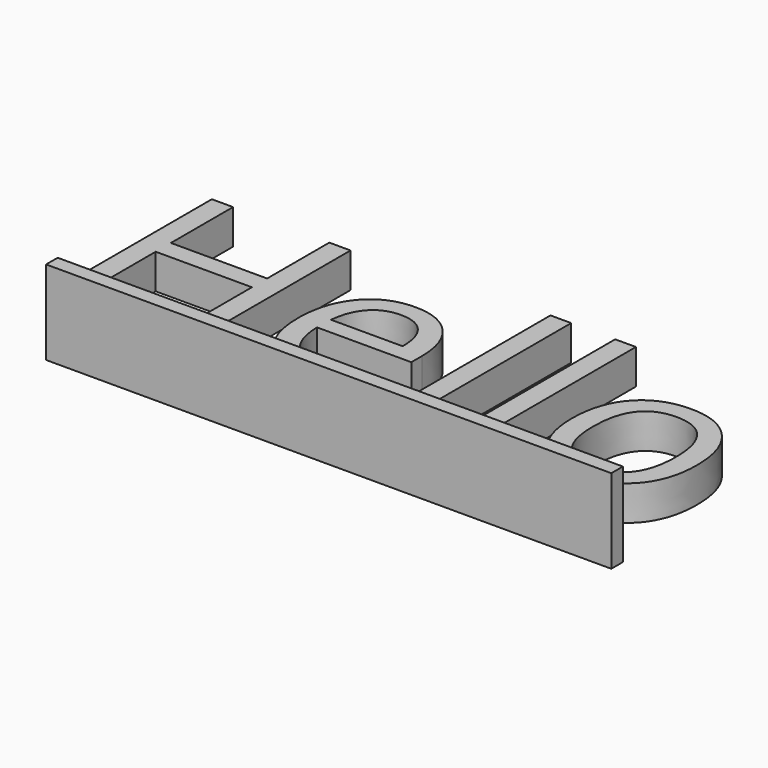
from build123d import *

# Parameters (mm, degrees)
F0_TEXT_SIZE = 55.8785550917
F1_DEPTH     = 7.62
F2_W         = 3.1644590199
F2_H         = 18.3762102388
F3_DEPTH     = 61.722


# Not quite as in the source:
# - Text() gives the source's letters only with a copy of the font that has no kerning and outlines rounded to 1/6400 em; it was checked with that copy


with BuildPart() as f1:
    # F0 (on Top) → F1 (new body)
    with BuildSketch(Plane.XY):
        with Locations((-65.4461756349, -20.6624232233)):
            Text('Hello', F0_TEXT_SIZE, font='Open Sans', text_align=(TextAlign.LEFT, TextAlign.BOTTOM))
    extrude(amount=F1_DEPTH)


with BuildPart() as f3:
    # F2 (on Right) → F3 (new body, symmetric)
    with BuildSketch(Plane.YZ):
        with Locations((-22.2446527332, 2.8249828611)):
            Rectangle(F2_W, F2_H)
    extrude(amount=F3_DEPTH, both=True)


solid = Compound([f1.part, f3.part])
